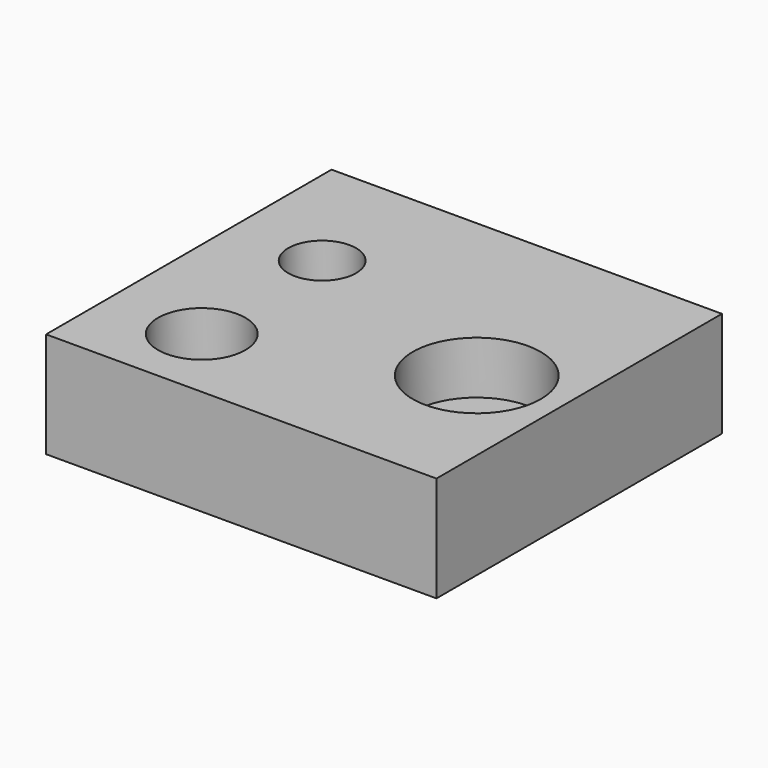
from build123d import *

# Parameters (mm, degrees)
F0_W     = 93.979999423
F0_H     = 85.8981758356
F1_DEPTH = 25.4
F2_R     = 10.5198846742
F2_R_2   = 8.1643500286
F2_R_3   = 15.4096343481
F3_DEPTH = 12.7


# Not quite as in the source:
# - a feature names something its author has since deleted; it is built from what else it names


with BuildPart() as f1:
    # F0 (on Top) → F1 (new body)
    with BuildSketch(Plane.XY):
        Rectangle(F0_W, F0_H)
    extrude(amount=F1_DEPTH)

    # F2 (on face) → F3 (cut)
    with BuildSketch(Plane.XY.offset(25.4)):
        with Locations((-24.2489445955, -24.5321765542)):
            Circle(F2_R)
        with Locations((-25.2142474055, 12.9084698856)):
            Circle(F2_R_2)
        with Locations((26.6870334744, -5.449811928)):
            Circle(F2_R_3)
    extrude(amount=-F3_DEPTH, mode=Mode.SUBTRACT)


solid = f1.part
